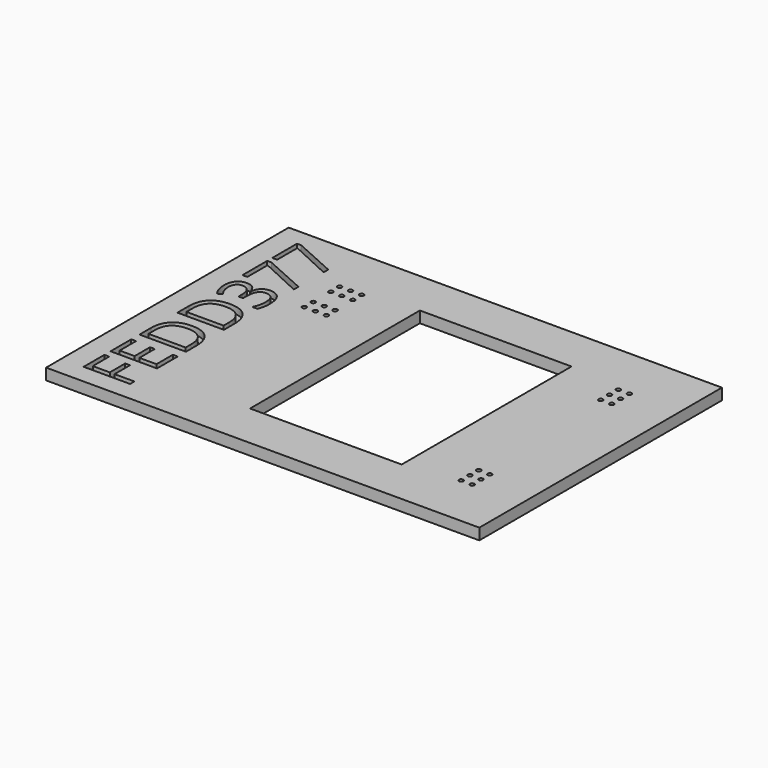
from build123d import *

# Parameters (mm, degrees)
F0_W         = 100
F0_H         = 70
F1_DEPTH     = 2.6
F2_TEXT_SIZE = 15.0251274715
F3_DEPTH     = 1.5
F4_W         = 35
F4_H         = 49
F4_R         = 0.5
F5_DEPTH     = 2.6


# Not quite as in the source:
# - Text() gives the source's letters only with a copy of the font that has no kerning and outlines rounded to 1/6400 em; it was checked with that copy


with BuildPart() as f1:
    # F0 (on Top) → F1 (new body)
    with BuildSketch(Plane.XY):
        with Locations((6.8412768841, 13.3350909071)):
            Rectangle(F0_W, F0_H)
    extrude(amount=F1_DEPTH)

    # F2 (on face) → F3 (cut)
    with BuildSketch(Plane.XY.offset(2.6)):
        with Locations(Location((-27.3406313365, -18.6649090929), (0, 0, 90))):
            Text('FEDD377', F2_TEXT_SIZE, font='Open Sans', text_align=(TextAlign.LEFT, TextAlign.BOTTOM))
    extrude(amount=-F3_DEPTH, mode=Mode.SUBTRACT)

    # F4 (on face) → F5 (cut, through all)
    with BuildSketch(Plane.XY.offset(2.6)):
        with Locations((13.0212768841, 13.3350909071)):
            Rectangle(F4_W, F4_H)
        with Locations((-21.5587231159, 36.0350909071)):
            Circle(F4_R)
        with Locations((-19.0187231159, 36.0350909071)):
            Circle(F4_R)
        with Locations((-16.4787231159, 36.0350909071)):
            Circle(F4_R)
        with Locations((-16.4787231159, 33.4950909071)):
            Circle(F4_R)
        with Locations((-16.4787231159, 28.3950909071)):
            Circle(F4_R)
        with Locations((-16.4787231159, 25.8550909071)):
            Circle(F4_R)
        with Locations((-19.0187231159, 25.8550909071)):
            Circle(F4_R)
        with Locations((-21.5587231159, 25.8550909071)):
            Circle(F4_R)
        with Locations((-21.5587231159, 28.3950909071)):
            Circle(F4_R)
        with Locations((-19.0187231159, 28.3950909071)):
            Circle(F4_R)
        with Locations((-19.0187231159, 33.4950909071)):
            Circle(F4_R)
        with Locations((-21.5587231159, 33.4950909071)):
            Circle(F4_R)
        with Locations((42.7712768841, -6.7849090929)):
            Circle(F4_R)
        with Locations((45.3112768841, -9.3249090929)):
            Circle(F4_R)
        with Locations((45.3112768841, -6.7849090929)):
            Circle(F4_R)
        with Locations((42.7712768841, -9.3249090929)):
            Circle(F4_R)
        with Locations((45.3112768841, -4.2449090929)):
            Circle(F4_R)
        with Locations((42.7712768841, -4.2449090929)):
            Circle(F4_R)
        with Locations((45.3112768841, 30.9550909071)):
            Circle(F4_R)
        with Locations((42.7712768841, 30.9550909071)):
            Circle(F4_R)
        with Locations((42.7712768841, 33.4950909071)):
            Circle(F4_R)
        with Locations((45.3112768841, 33.4950909071)):
            Circle(F4_R)
        with Locations((45.3112768841, 36.0350909071)):
            Circle(F4_R)
        with Locations((42.7712768841, 36.0350909071)):
            Circle(F4_R)
    extrude(amount=-F5_DEPTH, mode=Mode.SUBTRACT)


solid = f1.part
